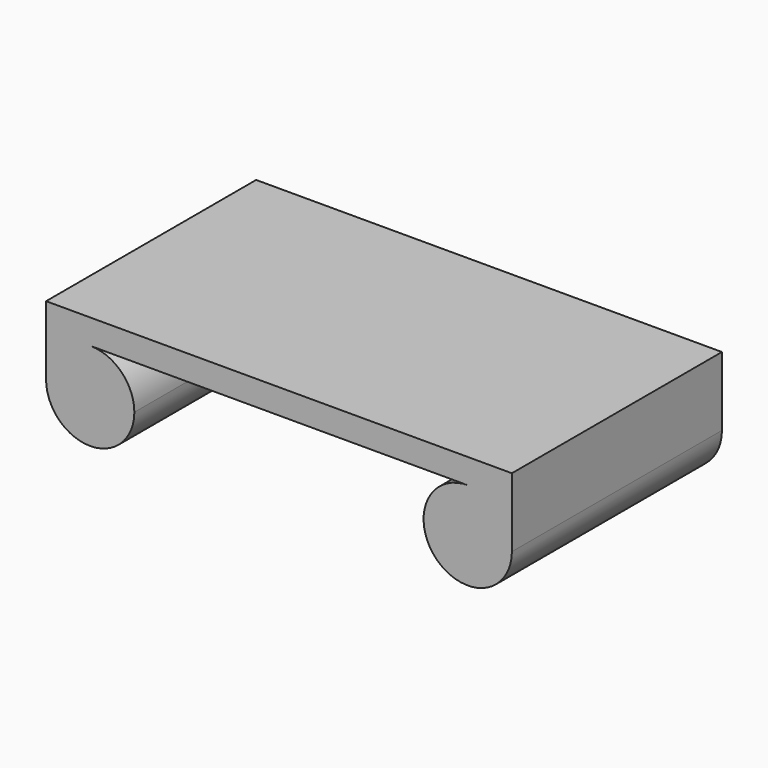
from build123d import *

# Parameters (mm, degrees)
F0_W     = 93.4585928917
F0_H     = 52.6832342148
F1_DEPTH = 5
F3_DEPTH = 52.6832342148


# Not quite as in the source:
# - a feature names something its author has since deleted; it is built from what else it names


with BuildPart() as f1:
    # F0 (on Top) → F1 (new body)
    with BuildSketch(Plane.XY):
        Rectangle(F0_W, F0_H)
    extrude(amount=F1_DEPTH)

    # F2 (on face) → F3 (join, through all)
    with BuildSketch(Plane.XZ.offset(26.3416171074)):
        with BuildLine():
            ThreePointArc((-46.7292964458, -8.8555142283), (-44.1355763793, -2.5937200666), (-37.8737822175, 0))
            Line((-37.8737822175, 0), (-46.7292964458, 0))
            Line((-46.7292964458, 0), (-46.7292964458, -8.8555142283))
        make_face()
        with BuildLine():
            ThreePointArc((46.7292964458, -8.8555142283), (44.1355763793, -2.5937200666), (37.8737822175, 0))
            ThreePointArc((37.8737822175, 0), (31.6119880557, -15.1173083901), (46.7292964458, -8.8555142283))
        make_face()
        with BuildLine():
            ThreePointArc((-46.7292964458, -8.8555142283), (-37.8737822175, -17.7110284567), (-29.0182679892, -8.8555142283))
            ThreePointArc((-29.0182679892, -8.8555142283), (-31.6119880557, -2.5937200666), (-37.8737822175, 0))
            ThreePointArc((-37.8737822175, 0), (-44.1355763793, -2.5937200666), (-46.7292964458, -8.8555142283))
        make_face()
        with BuildLine():
            Line((46.7292964458, 0), (37.8737822175, 0))
            ThreePointArc((37.8737822175, 0), (44.1355763793, -2.5937200666), (46.7292964458, -8.8555142283))
            Line((46.7292964458, -8.8555142283), (46.7292964458, 0))
        make_face()
    extrude(amount=-F3_DEPTH)


solid = f1.part
